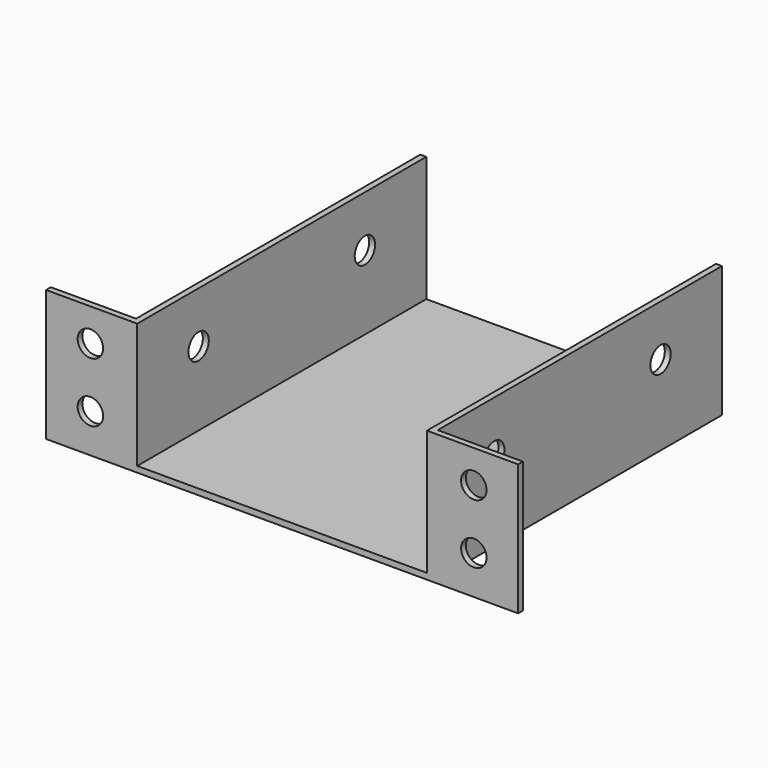
from build123d import *

# Parameters (mm, degrees)
F0_W     = 44.958
F0_H     = 53.848
F1_DEPTH = 0.889
F2_W     = 0.889
F2_H     = 18.669
F3_DEPTH = 53.848
F4_W     = 0.889
F4_H     = 19.558
F5_DEPTH = 12.7
F6_W     = 0.889
F6_H     = 19.558
F7_DEPTH = 12.7
F9_D     = 3.7973
F11_D    = 3.7973


# Not quite as in the source:
# - a feature names something its author has since deleted; it is built from what else it names


with BuildPart() as f1:
    # F0 (on Top) → F1 (new body)
    with BuildSketch(Plane.XY):
        with Locations((22.479, 26.924)):
            Rectangle(F0_W, F0_H)
    extrude(amount=F1_DEPTH)

    # F2 (on face) → F3 (join, through all)
    with BuildSketch(Plane.XZ):
        with Locations((0.4445, 10.2235)):
            Rectangle(F2_W, F2_H)
        with Locations((44.5135, 10.2235)):
            Rectangle(F2_W, F2_H)
    extrude(amount=-F3_DEPTH)

    # F4 (on face) → F5 (join)
    with BuildSketch(Plane(origin=(0, 0, 0), x_dir=(0, -1, 0), z_dir=(-1, 0, 0))):
        with Locations((-0.4445, 9.779)):
            Rectangle(F4_W, F4_H)
    extrude(amount=F5_DEPTH)

    # F6 (on face) → F7 (join)
    with BuildSketch(Plane.YZ.offset(44.958)):
        with Locations((0.4445, 9.779)):
            Rectangle(F6_W, F6_H)
    extrude(amount=F7_DEPTH)

    # F9 (through all)
    with Locations(Plane.XZ):
        with Locations((-6.096, 14.6685), (-6.096, 5.7785), (51.054, 5.7785), (51.054, 14.6685)):
            Hole(F9_D / 2)

    # F11 (through all)
    with Locations(Plane(origin=(0, 0, 0), x_dir=(0, -1, 0), z_dir=(-1, 0, 0))):
        with Locations((-11.43, 11.938), (-42.418, 11.938)):
            Hole(F11_D / 2)


solid = f1.part
